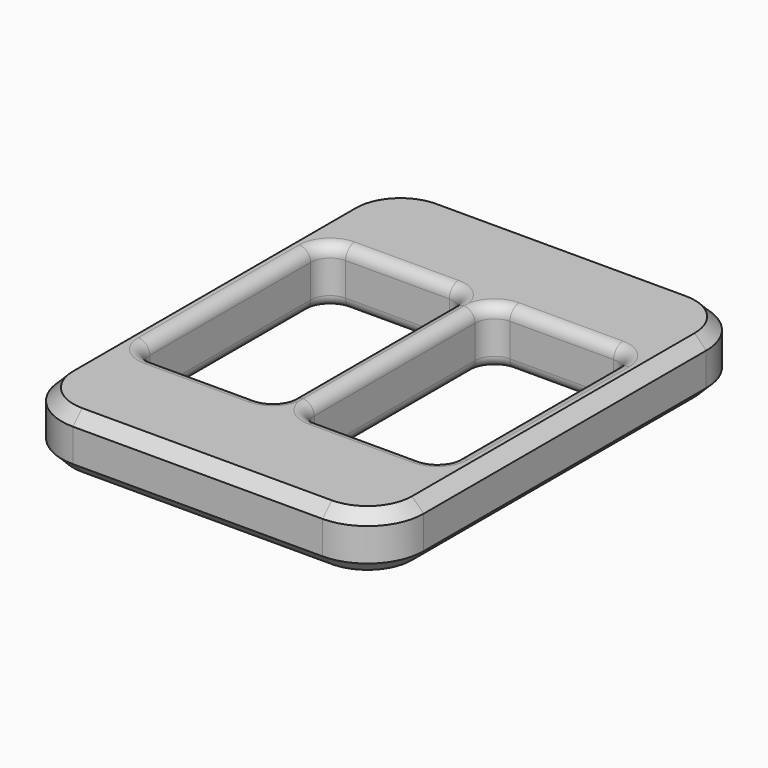
from build123d import *

# Parameters (mm, degrees)
F1_DEPTH     = 9.2202
F2_T1_DEPTH  = 32.9946
F2_T3_DEPTH  = 17.018
F2_T5_DEPTH  = 17.018
F2_T8_ANGLE  = 90
F2_T10_ANGLE = 90
F2_T12_ANGLE = 90
F2_T14_ANGLE = 90
F2_T16_ANGLE = 90
F2_T18_ANGLE = 90
F2_T20_ANGLE = 90
F2_T22_ANGLE = 90
F2_T24_ANGLE = 90
F2_T26_ANGLE = 90
F2_T28_ANGLE = 90
F2_T30_ANGLE = 90
F2_T32_ANGLE = 90
F2_T34_ANGLE = 90
F2_T36_ANGLE = 90
F2_T38_ANGLE = 90
F3_SIZE      = 1.905


# Not quite as in the source:
# - a fillet or chamfer that OpenCascade refuses, or shapes differently, is made with other operations: its cross-section is extruded or revolved along the edge and cut away or added


with BuildPart() as f1:
    # F0 (on Top) → F1 (new body)
    with BuildSketch(Plane.XY):
        with BuildLine():
            Line((20.4724, 76.4032), (-20.4724, 76.4032))
            ThreePointArc((-20.4724, 76.4032), (-26.9920659439, 73.7026659439), (-29.6926, 67.183))
            Line((-29.6926, 67.183), (-29.6926, 9.2202))
            ThreePointArc((-29.6926, 9.2202), (-26.9920659439, 2.7005340561), (-20.4724, 0))
            Line((-20.4724, 0), (20.4724, 0))
            ThreePointArc((20.4724, 0), (26.9920659439, 2.7005340561), (29.6926, 9.2202))
            Line((29.6926, 9.2202), (29.6926, 67.183))
            ThreePointArc((29.6926, 67.183), (26.9920659439, 73.7026659439), (20.4724, 76.4032))
        make_face()
        with BuildLine():
            Line((-25.1714, 21.6408), (-25.1714, 54.6354))
            ThreePointArc((-25.1714, 54.6354), (-24.2414640303, 56.8804640303), (-21.9964, 57.8104))
            Line((-21.9964, 57.8104), (-4.9784, 57.8104))
            ThreePointArc((-4.9784, 57.8104), (-2.7333359697, 56.8804640303), (-1.8034, 54.6354))
            Line((-1.8034, 54.6354), (-1.8034, 21.6408))
            ThreePointArc((-1.8034, 21.6408), (-2.7333359697, 19.3957359697), (-4.9784, 18.4658))
            Line((-4.9784, 18.4658), (-21.9964, 18.4658))
            ThreePointArc((-21.9964, 18.4658), (-24.2414640303, 19.3957359697), (-25.1714, 21.6408))
        make_face(mode=Mode.SUBTRACT)
        with BuildLine():
            Line((1.8034, 21.6408), (1.8034, 54.6354))
            ThreePointArc((1.8034, 54.6354), (2.7333359697, 56.8804640303), (4.9784, 57.8104))
            Line((4.9784, 57.8104), (21.9964, 57.8104))
            ThreePointArc((21.9964, 57.8104), (24.2414640303, 56.8804640303), (25.1714, 54.6354))
            Line((25.1714, 54.6354), (25.1714, 21.6408))
            ThreePointArc((25.1714, 21.6408), (24.2414640303, 19.3957359697), (21.9964, 18.4658))
            Line((21.9964, 18.4658), (4.9784, 18.4658))
            ThreePointArc((4.9784, 18.4658), (2.7333359697, 19.3957359697), (1.8034, 21.6408))
        make_face(mode=Mode.SUBTRACT)
    extrude(amount=F1_DEPTH)

    # F2: fillet of radius 1.905 on 4 edges, made by hand

    # F2_s2 → F2_t1 (cut)
    with BuildSketch(Plane.XZ.offset(-54.6354)):
        with BuildLine():
            ThreePointArc((25.1714, 1.905), (25.7293615818, 0.5579615818), (27.0764, 0))
            Line((27.0764, 0), (25.1714, 0))
            Line((25.1714, 0), (25.1714, 1.905))
        make_face()
        with BuildLine():
            ThreePointArc((-25.1714, 1.905), (-25.7293615818, 0.5579615818), (-27.0764, 0))
            Line((-27.0764, 0), (-25.1714, 0))
            Line((-25.1714, 0), (-25.1714, 1.905))
        make_face()
        with BuildLine():
            ThreePointArc((-1.8034, 7.3152), (-1.2454384182, 8.6622384182), (0.1016, 9.2202))
            Line((0.1016, 9.2202), (-1.8034, 9.2202))
            Line((-1.8034, 9.2202), (-1.8034, 7.3152))
        make_face()
        with BuildLine():
            ThreePointArc((25.1714, 7.3152), (25.7293615818, 8.6622384182), (27.0764, 9.2202))
            Line((27.0764, 9.2202), (25.1714, 9.2202))
            Line((25.1714, 9.2202), (25.1714, 7.3152))
        make_face()
        with BuildLine():
            ThreePointArc((1.8034, 7.3152), (1.2454384182, 8.6622384182), (-0.1016, 9.2202))
            Line((-0.1016, 9.2202), (1.8034, 9.2202))
            Line((1.8034, 9.2202), (1.8034, 7.3152))
        make_face()
        with BuildLine():
            ThreePointArc((-25.1714, 7.3152), (-25.7293615818, 8.6622384182), (-27.0764, 9.2202))
            Line((-27.0764, 9.2202), (-25.1714, 9.2202))
            Line((-25.1714, 9.2202), (-25.1714, 7.3152))
        make_face()
        with BuildLine():
            ThreePointArc((-1.8034, 1.905), (-1.2454384182, 0.5579615818), (0.1016, 0))
            Line((0.1016, 0), (-1.8034, 0))
            Line((-1.8034, 0), (-1.8034, 1.905))
        make_face()
        with BuildLine():
            ThreePointArc((1.8034, 1.905), (1.2454384182, 0.5579615818), (-0.1016, 0))
            Line((-0.1016, 0), (1.8034, 0))
            Line((1.8034, 0), (1.8034, 1.905))
        make_face()
    extrude(amount=F2_T1_DEPTH, mode=Mode.SUBTRACT)

    # F2_s4 → F2_t3 (cut)
    with BuildSketch(Plane.YZ.offset(4.9784)):
        with BuildLine():
            ThreePointArc((57.8104, 7.3152), (58.3683615818, 8.6622384182), (59.7154, 9.2202))
            Line((59.7154, 9.2202), (57.8104, 9.2202))
            Line((57.8104, 9.2202), (57.8104, 7.3152))
        make_face()
        with BuildLine():
            ThreePointArc((18.4658, 7.3152), (17.9078384182, 8.6622384182), (16.5608, 9.2202))
            Line((16.5608, 9.2202), (18.4658, 9.2202))
            Line((18.4658, 9.2202), (18.4658, 7.3152))
        make_face()
        with BuildLine():
            ThreePointArc((18.4658, 1.905), (17.9078384182, 0.5579615818), (16.5608, 0))
            Line((16.5608, 0), (18.4658, 0))
            Line((18.4658, 0), (18.4658, 1.905))
        make_face()
        with BuildLine():
            ThreePointArc((57.8104, 1.905), (58.3683615818, 0.5579615818), (59.7154, 0))
            Line((59.7154, 0), (57.8104, 0))
            Line((57.8104, 0), (57.8104, 1.905))
        make_face()
    extrude(amount=F2_T3_DEPTH, mode=Mode.SUBTRACT)

    # F2_s6 → F2_t5 (cut)
    with BuildSketch(Plane.YZ.offset(-21.9964)):
        with BuildLine():
            ThreePointArc((18.4658, 7.3152), (17.9078384182, 8.6622384182), (16.5608, 9.2202))
            Line((16.5608, 9.2202), (18.4658, 9.2202))
            Line((18.4658, 9.2202), (18.4658, 7.3152))
        make_face()
        with BuildLine():
            ThreePointArc((57.8104, 7.3152), (58.3683615818, 8.6622384182), (59.7154, 9.2202))
            Line((59.7154, 9.2202), (57.8104, 9.2202))
            Line((57.8104, 9.2202), (57.8104, 7.3152))
        make_face()
        with BuildLine():
            ThreePointArc((57.8104, 1.905), (58.3683615818, 0.5579615818), (59.7154, 0))
            Line((59.7154, 0), (57.8104, 0))
            Line((57.8104, 0), (57.8104, 1.905))
        make_face()
        with BuildLine():
            ThreePointArc((18.4658, 1.905), (17.9078384182, 0.5579615818), (16.5608, 0))
            Line((16.5608, 0), (18.4658, 0))
            Line((18.4658, 0), (18.4658, 1.905))
        make_face()
    extrude(amount=F2_T5_DEPTH, mode=Mode.SUBTRACT)

    # F2_s7 → F2_t8 (revolve, cut)
    with BuildSketch(Plane.XZ.offset(-54.6354)):
        with BuildLine():
            ThreePointArc((1.8034, 7.3152), (1.2454384182, 8.6622384182), (-0.1016, 9.2202))
            Line((-0.1016, 9.2202), (1.8034, 9.2202))
            Line((1.8034, 9.2202), (1.8034, 7.3152))
        make_face()
    revolve(axis=Axis((4.9784, 54.6354, 9.2202), (0, 0, -1)), revolution_arc=F2_T8_ANGLE, mode=Mode.SUBTRACT)

    # F2_s9 → F2_t10 (revolve, cut)
    with BuildSketch(Plane.YZ.offset(21.9964)):
        with BuildLine():
            ThreePointArc((57.8104, 7.3152), (58.3683615818, 8.6622384182), (59.7154, 9.2202))
            Line((59.7154, 9.2202), (57.8104, 9.2202))
            Line((57.8104, 9.2202), (57.8104, 7.3152))
        make_face()
    revolve(axis=Axis((21.9964, 54.6354, 9.2202), (0, 0, -1)), revolution_arc=F2_T10_ANGLE, mode=Mode.SUBTRACT)

    # F2_s11 → F2_t12 (revolve, cut)
    with BuildSketch(Plane.XZ.offset(-21.6408)):
        with BuildLine():
            ThreePointArc((25.1714, 7.3152), (25.7293615818, 8.6622384182), (27.0764, 9.2202))
            Line((27.0764, 9.2202), (25.1714, 9.2202))
            Line((25.1714, 9.2202), (25.1714, 7.3152))
        make_face()
    revolve(axis=Axis((21.9964, 21.6408, 9.2202), (0, 0, -1)), revolution_arc=F2_T12_ANGLE, mode=Mode.SUBTRACT)

    # F2_s13 → F2_t14 (revolve, cut)
    with BuildSketch(Plane.YZ.offset(4.9784)):
        with BuildLine():
            ThreePointArc((18.4658, 7.3152), (17.9078384182, 8.6622384182), (16.5608, 9.2202))
            Line((16.5608, 9.2202), (18.4658, 9.2202))
            Line((18.4658, 9.2202), (18.4658, 7.3152))
        make_face()
    revolve(axis=Axis((4.9784, 21.6408, 9.2202), (0, 0, -1)), revolution_arc=F2_T14_ANGLE, mode=Mode.SUBTRACT)

    # F2_s15 → F2_t16 (revolve, cut)
    with BuildSketch(Plane.YZ.offset(-4.9784)):
        with BuildLine():
            ThreePointArc((57.8104, 7.3152), (58.3683615818, 8.6622384182), (59.7154, 9.2202))
            Line((59.7154, 9.2202), (57.8104, 9.2202))
            Line((57.8104, 9.2202), (57.8104, 7.3152))
        make_face()
    revolve(axis=Axis((-4.9784, 54.6354, 9.2202), (0, 0, -1)), revolution_arc=F2_T16_ANGLE, mode=Mode.SUBTRACT)

    # F2_s17 → F2_t18 (revolve, cut)
    with BuildSketch(Plane.XZ.offset(-21.6408)):
        with BuildLine():
            ThreePointArc((-1.8034, 7.3152), (-1.2454384182, 8.6622384182), (0.1016, 9.2202))
            Line((0.1016, 9.2202), (-1.8034, 9.2202))
            Line((-1.8034, 9.2202), (-1.8034, 7.3152))
        make_face()
    revolve(axis=Axis((-4.9784, 21.6408, 9.2202), (0, 0, -1)), revolution_arc=F2_T18_ANGLE, mode=Mode.SUBTRACT)

    # F2_s19 → F2_t20 (revolve, cut)
    with BuildSketch(Plane.YZ.offset(-21.9964)):
        with BuildLine():
            ThreePointArc((18.4658, 7.3152), (17.9078384182, 8.6622384182), (16.5608, 9.2202))
            Line((16.5608, 9.2202), (18.4658, 9.2202))
            Line((18.4658, 9.2202), (18.4658, 7.3152))
        make_face()
    revolve(axis=Axis((-21.9964, 21.6408, 9.2202), (0, 0, -1)), revolution_arc=F2_T20_ANGLE, mode=Mode.SUBTRACT)

    # F2_s21 → F2_t22 (revolve, cut)
    with BuildSketch(Plane.XZ.offset(-54.6354)):
        with BuildLine():
            ThreePointArc((-25.1714, 7.3152), (-25.7293615818, 8.6622384182), (-27.0764, 9.2202))
            Line((-27.0764, 9.2202), (-25.1714, 9.2202))
            Line((-25.1714, 9.2202), (-25.1714, 7.3152))
        make_face()
    revolve(axis=Axis((-21.9964, 54.6354, 9.2202), (0, 0, -1)), revolution_arc=F2_T22_ANGLE, mode=Mode.SUBTRACT)

    # F2_s23 → F2_t24 (revolve, cut)
    with BuildSketch(Plane.YZ.offset(-21.9964)):
        with BuildLine():
            ThreePointArc((18.4658, 1.905), (17.9078384182, 0.5579615818), (16.5608, 0))
            Line((16.5608, 0), (18.4658, 0))
            Line((18.4658, 0), (18.4658, 1.905))
        make_face()
    revolve(axis=Axis((-21.9964, 21.6408, 0), (0, 0, -1)), revolution_arc=F2_T24_ANGLE, mode=Mode.SUBTRACT)

    # F2_s25 → F2_t26 (revolve, cut)
    with BuildSketch(Plane.XZ.offset(-54.6354)):
        with BuildLine():
            ThreePointArc((-25.1714, 1.905), (-25.7293615818, 0.5579615818), (-27.0764, 0))
            Line((-27.0764, 0), (-25.1714, 0))
            Line((-25.1714, 0), (-25.1714, 1.905))
        make_face()
    revolve(axis=Axis((-21.9964, 54.6354, 0), (0, 0, -1)), revolution_arc=F2_T26_ANGLE, mode=Mode.SUBTRACT)

    # F2_s27 → F2_t28 (revolve, cut)
    with BuildSketch(Plane.YZ.offset(-4.9784)):
        with BuildLine():
            ThreePointArc((57.8104, 1.905), (58.3683615818, 0.5579615818), (59.7154, 0))
            Line((59.7154, 0), (57.8104, 0))
            Line((57.8104, 0), (57.8104, 1.905))
        make_face()
    revolve(axis=Axis((-4.9784, 54.6354, 0), (0, 0, -1)), revolution_arc=F2_T28_ANGLE, mode=Mode.SUBTRACT)

    # F2_s29 → F2_t30 (revolve, cut)
    with BuildSketch(Plane.XZ.offset(-21.6408)):
        with BuildLine():
            ThreePointArc((-1.8034, 1.905), (-1.2454384182, 0.5579615818), (0.1016, 0))
            Line((0.1016, 0), (-1.8034, 0))
            Line((-1.8034, 0), (-1.8034, 1.905))
        make_face()
    revolve(axis=Axis((-4.9784, 21.6408, 0), (0, 0, -1)), revolution_arc=F2_T30_ANGLE, mode=Mode.SUBTRACT)

    # F2_s31 → F2_t32 (revolve, cut)
    with BuildSketch(Plane.YZ.offset(21.9964)):
        with BuildLine():
            ThreePointArc((57.8104, 1.905), (58.3683615818, 0.5579615818), (59.7154, 0))
            Line((59.7154, 0), (57.8104, 0))
            Line((57.8104, 0), (57.8104, 1.905))
        make_face()
    revolve(axis=Axis((21.9964, 54.6354, 0), (0, 0, -1)), revolution_arc=F2_T32_ANGLE, mode=Mode.SUBTRACT)

    # F2_s33 → F2_t34 (revolve, cut)
    with BuildSketch(Plane.XZ.offset(-21.6408)):
        with BuildLine():
            ThreePointArc((25.1714, 1.905), (25.7293615818, 0.5579615818), (27.0764, 0))
            Line((27.0764, 0), (25.1714, 0))
            Line((25.1714, 0), (25.1714, 1.905))
        make_face()
    revolve(axis=Axis((21.9964, 21.6408, 0), (0, 0, -1)), revolution_arc=F2_T34_ANGLE, mode=Mode.SUBTRACT)

    # F2_s35 → F2_t36 (revolve, cut)
    with BuildSketch(Plane.YZ.offset(4.9784)):
        with BuildLine():
            ThreePointArc((18.4658, 1.905), (17.9078384182, 0.5579615818), (16.5608, 0))
            Line((16.5608, 0), (18.4658, 0))
            Line((18.4658, 0), (18.4658, 1.905))
        make_face()
    revolve(axis=Axis((4.9784, 21.6408, 0), (0, 0, -1)), revolution_arc=F2_T36_ANGLE, mode=Mode.SUBTRACT)

    # F2_s37 → F2_t38 (revolve, cut)
    with BuildSketch(Plane.XZ.offset(-54.6354)):
        with BuildLine():
            ThreePointArc((1.8034, 1.905), (1.2454384182, 0.5579615818), (-0.1016, 0))
            Line((-0.1016, 0), (1.8034, 0))
            Line((1.8034, 0), (1.8034, 1.905))
        make_face()
    revolve(axis=Axis((4.9784, 54.6354, 0), (0, 0, -1)), revolution_arc=F2_T38_ANGLE, mode=Mode.SUBTRACT)

    # F3
    f3_edges = [f1.edges().sort_by_distance(p)[0] for p in [
        (-29.6926, 38.2016, 9.2202),
        (-29.6926, 38.2016, 0),
    ]]
    chamfer(f3_edges, length=F3_SIZE)


solid = f1.part
